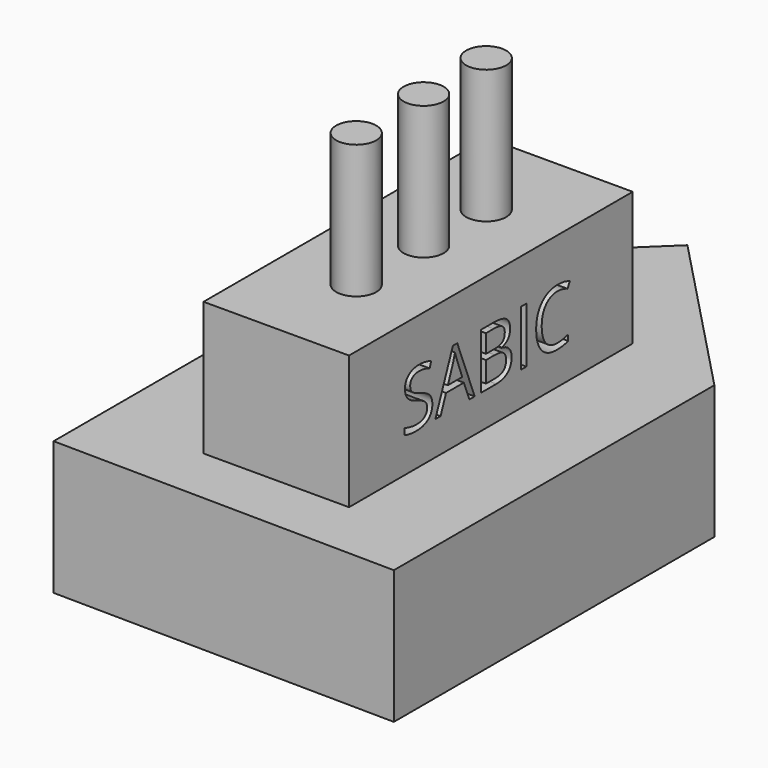
from build123d import *

# Parameters (mm, degrees)
F1_DEPTH     = 25.4
F2_W         = 27.6673045009
F2_H         = 67.4390569329
F3_DEPTH     = 25.4
F4_R         = 3.81
F5_DEPTH     = 25.4
F6_TEXT_SIZE = 14.7900181926
F7_DEPTH     = 63.5


# Not quite as in the source:
# - Text() gives the source's letters only with a copy of the font that has no kerning and outlines rounded to 1/6400 em; it was checked with that copy


with BuildPart() as f1:
    # F0 (on Top) → F1 (new body)
    with BuildSketch(Plane.XY):
        Polygon((31.2546874716, 43.7521982265), (0, 76.4093399224), (-34.1225265718, 43.7521982265), (-34.1225265718, -31.6104366647), (31.2546874716, -32.4478017735), align=None)
    extrude(amount=F1_DEPTH)

    # F2 (on face) → F3 (join)
    with BuildSketch(Plane.XY.offset(25.4)):
        with Locations((-0.432302244, 12.9296183586)):
            Rectangle(F2_W, F2_H)
    extrude(amount=F3_DEPTH)

    # F4 (on face) → F5 (join)
    with BuildSketch(Plane.XY.offset(50.8)):
        with Locations((0, 28.5708817181)):
            Circle(F4_R)
        with Locations((0, 13.6977448858)):
            Circle(F4_R)
        with Locations((0, -2.3194812864)):
            Circle(F4_R)
    extrude(amount=F5_DEPTH)

    # F6 (on face) → F7 (cut)
    with BuildSketch(Plane.YZ.offset(13.4013500065)):
        with Locations((-8.3856014535, 31.8025350571)):
            Text('SABIC', F6_TEXT_SIZE, font='Open Sans', text_align=(TextAlign.LEFT, TextAlign.BOTTOM))
    extrude(amount=-F7_DEPTH, mode=Mode.SUBTRACT)


solid = f1.part
